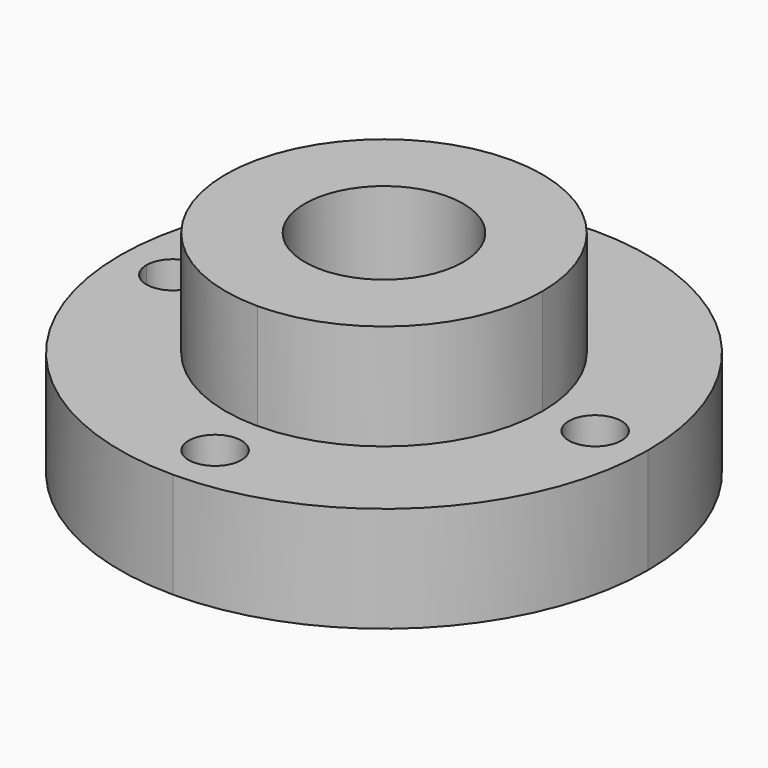
from build123d import *

# Parameters (mm, degrees)
F0_W     = 63.5
F0_H     = 63.5
F1_DEPTH = 25.4
F2_W     = 63.5
F2_H     = 63.5
F3_DEPTH = 12.7
F5_DEPTH = 25.4
F7_DEPTH = 25.4
F8_R     = 31.74999
F9_R     = 19.04999


# Not quite as in the source:
# - a fillet or chamfer is up to 0.001 mm smaller than in the source, because OpenCascade refuses the exact size


with BuildPart() as f1:
    # F0 (on Top) → F1 (new body)
    with BuildSketch(Plane.XY):
        with Locations((31.75, 31.75)):
            Rectangle(F0_W, F0_H)
    extrude(amount=F1_DEPTH)

    # F2 (on face) → F3 (cut)
    with BuildSketch(Plane.XY.offset(25.4)):
        with Locations((31.75, 31.75)):
            Rectangle(F2_W, F2_H)
        Polygon((12.7, 50.8), (31.75, 50.8), (50.8, 50.8), (50.8, 31.75), (50.8, 12.7), (12.7, 12.7), align=None, mode=Mode.SUBTRACT)
    extrude(amount=-F3_DEPTH, mode=Mode.SUBTRACT)

    # F4 (on face) → F5 (cut)
    with BuildSketch(Plane.XY.offset(12.7)):
        with BuildLine():
            ThreePointArc((8.333406776, 34.22925847), (4.9746257807, 34.6116377753), (3.175, 31.75))
            Line((3.175, 31.75), (6.35, 31.75))
            Line((6.35, 31.75), (8.333406776, 34.22925847))
        make_face()
        with BuildLine():
            ThreePointArc((34.925, 57.15), (33.9950640303, 59.3950640303), (31.75, 60.325))
            ThreePointArc((31.75, 60.325), (29.5049359697, 54.9049359697), (34.925, 57.15))
        make_face()
        with BuildLine():
            Line((6.35, 31.75), (3.175, 31.75))
            ThreePointArc((3.175, 31.75), (6.35, 28.575), (9.525, 31.75))
            ThreePointArc((9.525, 31.75), (9.2116377753, 33.1253742193), (8.333406776, 34.22925847))
            Line((8.333406776, 34.22925847), (6.35, 31.75))
        make_face()
        with BuildLine():
            ThreePointArc((55.166593224, 29.27074153), (58.5253742193, 28.8883622247), (60.325, 31.75))
            Line((60.325, 31.75), (57.15, 31.75))
            Line((57.15, 31.75), (55.166593224, 29.27074153))
        make_face()
        with BuildLine():
            Line((57.15, 31.75), (60.325, 31.75))
            ThreePointArc((60.325, 31.75), (55.7746257807, 34.6116377753), (55.166593224, 29.27074153))
            Line((55.166593224, 29.27074153), (57.15, 31.75))
        make_face()
        with BuildLine():
            ThreePointArc((34.925, 6.35), (29.5049359697, 8.5950640303), (31.75, 3.175))
            ThreePointArc((31.75, 3.175), (33.9950640303, 4.1049359697), (34.925, 6.35))
        make_face()
    extrude(amount=-F5_DEPTH, mode=Mode.SUBTRACT)

    # F6 (on face) → F7 (cut)
    with BuildSketch(Plane.XY.offset(25.4)):
        with BuildLine():
            ThreePointArc((41.275, 31.75), (38.4851920908, 38.4851920908), (31.75, 41.275))
            Line((31.75, 41.275), (31.75, 22.225))
            ThreePointArc((31.75, 22.225), (38.4851920908, 25.0148079092), (41.275, 31.75))
        make_face()
        with BuildLine():
            Line((31.75, 22.225), (31.75, 41.275))
            ThreePointArc((31.75, 41.275), (22.225, 31.75), (31.75, 22.225))
        make_face()
    extrude(amount=-F7_DEPTH, mode=Mode.SUBTRACT)

    # F8 (radius 31.75 in the source; OpenCascade refuses exactly that, so slightly less here)
    f8_edges = [f1.edges().sort_by_distance(p)[0] for p in [
        (0, 0, 6.35),
        (63.5, 0, 6.35),
        (63.5, 63.5, 6.35),
        (0, 63.5, 6.35),
    ]]
    fillet(f8_edges, radius=F8_R)

    # F9 (radius 19.05 in the source; OpenCascade refuses exactly that, so slightly less here)
    f9_edges = [f1.edges().sort_by_distance(p)[0] for p in [
        (12.7, 12.7, 19.05),
        (50.8, 12.7, 19.05),
        (12.7, 50.8, 19.05),
        (50.8, 50.8, 19.05),
    ]]
    fillet(f9_edges, radius=F9_R)


solid = f1.part
